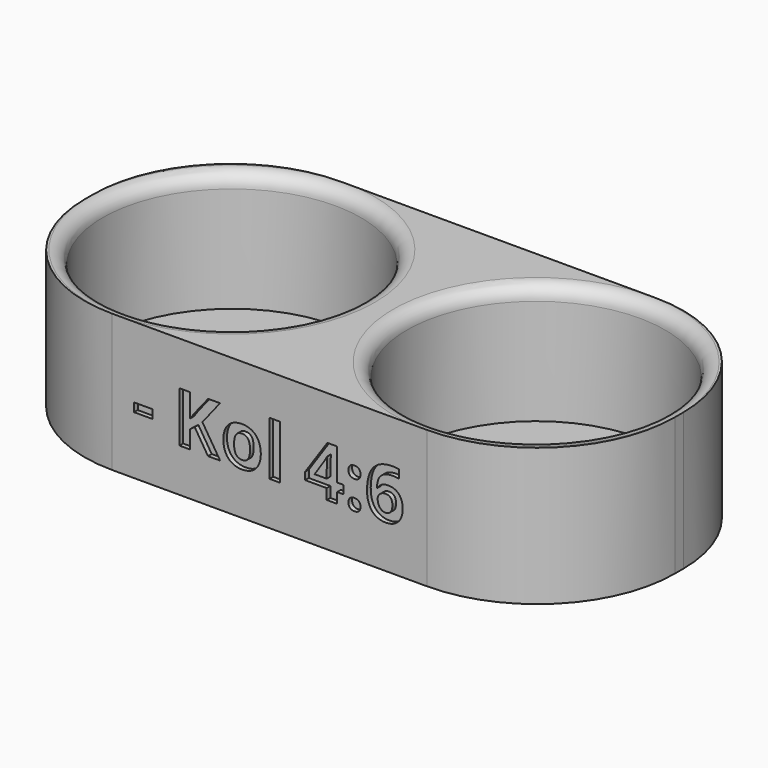
from build123d import *

# Parameters (mm, degrees)
F0_W         = 128.6
F0_H         = 62.3
F0_R         = 28.15
F1_DEPTH     = 30
F2_DEPTH     = 4
F3_R         = 30
F4_R         = 2.99999
F5_TEXT_SIZE = 15.4254037117
F6_DEPTH     = 1


# Not quite as in the source:
# - a fillet or chamfer is up to 0.001 mm smaller than in the source, because OpenCascade refuses the exact size
# - Text() gives the source's letters only with a copy of the font that has no kerning and outlines rounded to 1/6400 em; it was checked with that copy


with BuildPart() as f1:
    # F0 (on Top) → F1 (new body)
    with BuildSketch(Plane.XY):
        Rectangle(F0_W, F0_H)
        with Locations((-33.15, 0)):
            Circle(F0_R, mode=Mode.SUBTRACT)
        with Locations((33.15, 0)):
            Circle(F0_R, mode=Mode.SUBTRACT)
    extrude(amount=F1_DEPTH)

    # F0 (on Top) → F2 (join)
    with BuildSketch(Plane.XY):
        with Locations((-33.15, 0)):
            Circle(F0_R)
        with Locations((33.15, 0)):
            Circle(F0_R)
    extrude(amount=F2_DEPTH)

    # F3
    f3_edges = [f1.edges().sort_by_distance(p)[0] for p in [
        (-64.3, 31.15, 15),
        (-64.3, -31.15, 15),
        (64.3, -31.15, 15),
        (64.3, 31.15, 15),
    ]]
    fillet(f3_edges, radius=F3_R)

    # F4 (radius 3 in the source; OpenCascade refuses exactly that, so slightly less here)
    f4_edges = [f1.edges().sort_by_distance(p)[0] for p in [
        (-61.3, 0, 30),
        (5, 0, 30),
    ]]
    fillet(f4_edges, radius=F4_R)

    # F5 (on face) → F6 (cut)
    with BuildSketch(Plane.XZ.offset(31.15)):
        with Locations((-30, 9.4537093275)):
            Text('- Kol 4:6', F5_TEXT_SIZE, font='Open Sans', font_style=FontStyle.BOLD, text_align=(TextAlign.LEFT, TextAlign.BOTTOM))
    extrude(amount=-F6_DEPTH, mode=Mode.SUBTRACT)


solid = f1.part
